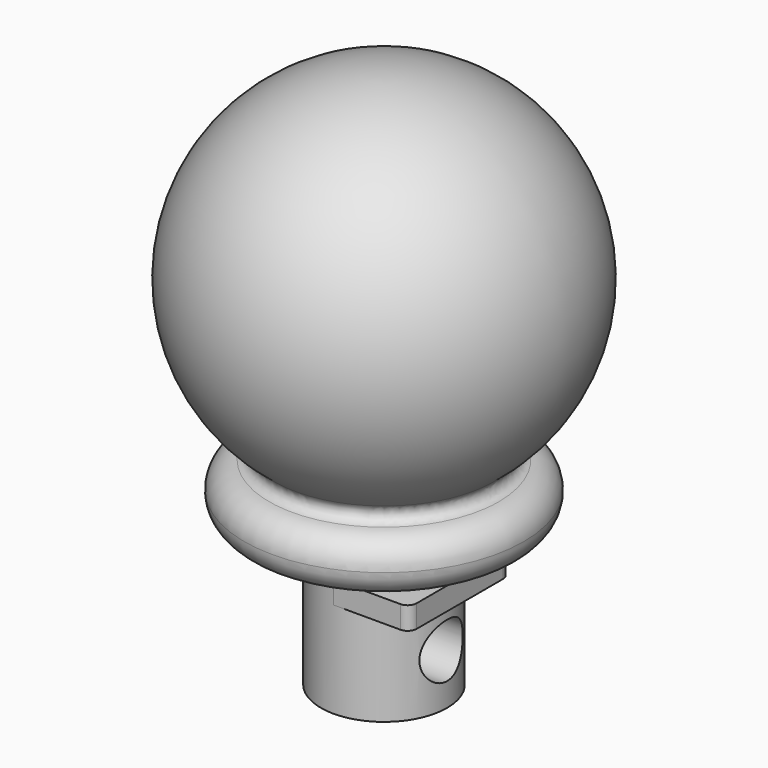
from build123d import *

# Parameters (mm, degrees)
F3_DEPTH = 2.5
F5_DEPTH = 13
F6_R     = 2.99999
F7_R     = 1
F8_R     = 1
F9_R     = 0.5


# Not quite as in the source:
# - a fillet or chamfer is up to 0.001 mm smaller than in the source, because OpenCascade refuses the exact size


with BuildPart() as f1:
    # F0 (on Front) → F1 (revolve)
    with BuildSketch(Plane.XZ):
        with BuildLine():
            Line((0, 59.8), (0, 0))
            Line((0, 0), (7, 0))
            Line((7, 0), (7, 13.12))
            Line((7, 13.12), (4.925, 13.12))
            Line((4.925, 13.12), (4.925, 16))
            Line((4.925, 16), (15.5, 16))
            Line((15.5, 16), (15.5, 22))
            Line((15.5, 22), (9.4249668434, 22))
            ThreePointArc((9.4249668434, 22), (19.4786421498, 44.5817607518), (0, 59.8))
        make_face()
    revolve(axis=Axis((0, 0, 29.9), (0, 0, 1)))

    # F2 (on face) → F3 (join)
    with BuildSketch(Plane.XY.offset(13.12)):
        with BuildLine():
            ThreePointArc((0, 7), (7, 0), (0, -7))
            Line((0, -7), (8.42, -7))
            Line((8.42, -7), (8.42, 7))
            Line((8.42, 7), (0, 7))
        make_face()
    extrude(amount=-F3_DEPTH)

    # F4 (on face) → F5 (cut)
    with BuildSketch(Plane.YZ.offset(8.42)):
        with BuildLine():
            ThreePointArc((-3, 5.62), (0, 2.62), (3, 5.62))
            Line((3, 5.62), (-3, 5.62))
        make_face()
        with BuildLine():
            Line((-3, 5.62), (3, 5.62))
            ThreePointArc((3, 5.62), (0, 8.62), (-3, 5.62))
        make_face()
    extrude(amount=-F5_DEPTH, mode=Mode.SUBTRACT)

    # F6 (radius 3 in the source; OpenCascade refuses exactly that, so slightly less here)
    f6_edges = [f1.edges().sort_by_distance(p)[0] for p in [
        (-15.5, 0, 22),
        (-15.5, 0, 16),
    ]]
    fillet(f6_edges, radius=F6_R)

    # F7
    f7_edges = [f1.edges().sort_by_distance(p)[0] for p in [
        (-9.424967, 0, 22),
    ]]
    fillet(f7_edges, radius=F7_R)

    # F8
    f8_edges = [f1.edges().sort_by_distance(p)[0] for p in [
        (8.42, -7, 11.87),
        (8.42, 7, 11.87),
    ]]
    fillet(f8_edges, radius=F8_R)

    # F9
    f9_edges = [f1.edges().sort_by_distance(p)[0] for p in [
        (-4.925, 0, 16),
    ]]
    fillet(f9_edges, radius=F9_R)


solid = f1.part
